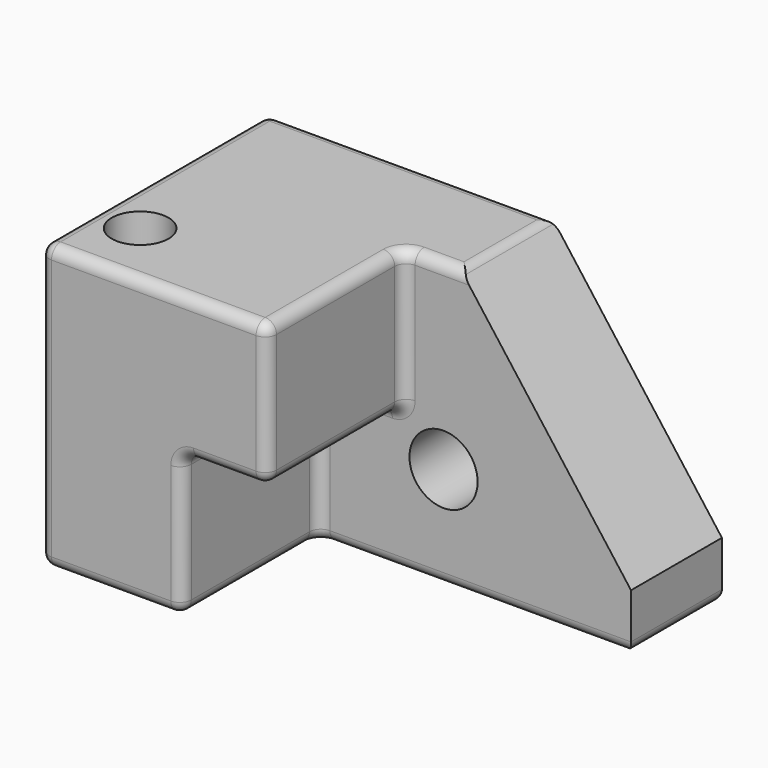
from build123d import *

# Parameters (mm, degrees)
F0_W     = 203.2
F0_H     = 127
F1_DEPTH = 127
F3_DEPTH = 76.2
F4_SIZE2 = 101.6
F4_SIZE  = 76.2
F5_R     = 5.08
F6_R     = 15.24
F7_DEPTH = 50.8
F8_R     = 12.7
F9_DEPTH = 127


with BuildPart() as f1:
    # F0 (on Front) → F1 (new body)
    with BuildSketch(Plane.XZ):
        with Locations((0.9113103151, -4.8755629536)):
            Rectangle(F0_W, F0_H)
    extrude(amount=F1_DEPTH)

    # F2 (on face) → F3 (cut)
    with BuildSketch(Plane.XZ.offset(127)):
        Polygon((102.5113103151, 58.6244370464), (0.9113103151, 58.6244370464), (0.9113103151, -4.8755629536), (-37.1886896849, -4.8755629536), (-37.1886896849, -68.3755629536), (102.5113103151, -68.3755629536), align=None)
    extrude(amount=-F3_DEPTH, mode=Mode.SUBTRACT)

    # F4
    f4_edges = [f1.edges().sort_by_distance(p)[0] for p in [
        (102.51131, -25.4, 58.624437),
    ]]
    f4_side = f1.faces().sort_by_distance((-20.860118, -52.614286, 58.624437))[0]
    chamfer(f4_edges, length=F4_SIZE, length2=F4_SIZE2, reference=f4_side)

    # F5
    f5_edges = [f1.edges().sort_by_distance(p)[0] for p in [
        (0.91131, -88.9, 58.624437),
        (26.31131, -25.4, 58.624437),
        (13.61131, -50.8, 58.624437),
        (-49.88869, -127, 58.624437),
        (0.91131, -127, 26.874437),
        (0.91131, -88.9, -4.875563),
        (-18.13869, -127, -4.875563),
        (-37.18869, -127, -36.625563),
        (32.66131, -50.8, -68.375563),
        (-37.18869, -88.9, -68.375563),
        (-68.93869, -127, -68.375563),
        (-100.68869, -127, -4.875563),
        (-100.68869, -63.5, 58.624437),
        (-37.18869, 0, 58.624437),
        (102.51131, -25.4, -68.375563),
        (-100.68869, 0, -4.875563),
        (-100.68869, -63.5, -68.375563),
        (0.91131, 0, -68.375563),
        (0.91131, -50.8, 26.874437),
        (-37.18869, -50.8, -36.625563),
        (-37.18869, -88.9, -4.875563),
        (-18.13869, -50.8, -4.875563),
    ]]
    fillet(f5_edges, radius=F5_R)

    # F6 (on face) → F7 (cut, through all)
    with BuildSketch(Plane.XZ.offset(50.8)):
        with Locations((18.6913103151, -22.6555629536)):
            Circle(F6_R)
    extrude(amount=-F7_DEPTH, mode=Mode.SUBTRACT)

    # F8 (on face) → F9 (cut, through all)
    with BuildSketch(Plane.XY.offset(58.6244370464)):
        with Locations((-80.3686896849, -96.52)):
            Circle(F8_R)
    extrude(amount=-F9_DEPTH, mode=Mode.SUBTRACT)


solid = f1.part
